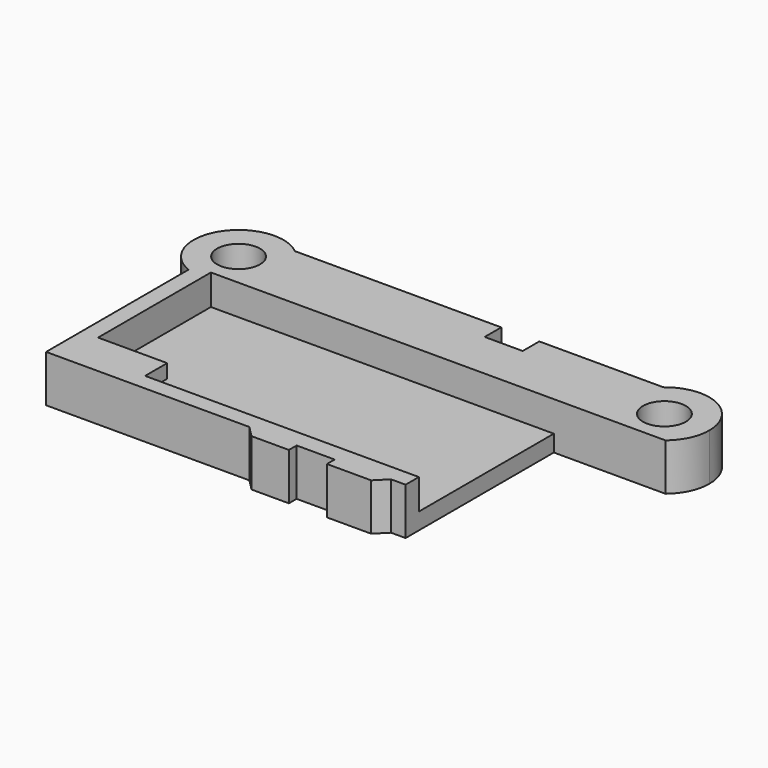
from build123d import *

# Parameters (mm, degrees)
F0_W        = 21.3
F0_H        = 2.5
F0_R        = 1.55
F1_DEPTH    = 3.4
F0_W_2      = 1.2
F0_H_2      = 1.2
F0_W_3      = 3.5
F2_DEPTH    = 3.4
F0_H_3      = 12.2
F3_DEPTH    = 1.2
F4_W        = 5
F4_H        = 1
F5_DEPTH    = 2
F6_T4_DEPTH = 3.4
F6_T9_DEPTH = 3.4


# Not quite as in the source:
# - a fillet or chamfer that OpenCascade refuses, or shapes differently, is made with other operations: its cross-section is extruded or revolved along the edge and cut away or added
# - a feature names something its author has since deleted; it is built from what else it names


with BuildPart() as f1:
    # F0 (on Top) → F1 (new body)
    with BuildSketch(Plane.XY):
        with BuildLine():
            ThreePointArc((-16.4319353276, -0.9810708435), (-15.752751994, 1.4598801321), (-13.6819353276, 0))
            ThreePointArc((-13.6819353276, 0), (-14.1359198167, -1.0960155108), (-15.2319353276, -1.55))
            Line((-15.2319353276, -1.55), (-15.2319353276, -2.5))
            Line((-15.2319353276, -2.5), (-13.1552793618, -2.5))
            ThreePointArc((-13.1552793618, -2.5), (-12.2898585195, -1.3808273084), (-11.9819353276, 0))
            ThreePointArc((-11.9819353276, 0), (-12.2898585195, 1.3808273084), (-13.1552793618, 2.5))
            ThreePointArc((-13.1552793618, 2.5), (-18.0266966766, 1.6588577401), (-16.4319353276, -3.0203476621))
            Line((-16.4319353276, -3.0203476621), (-16.4319353276, -2.5))
            Line((-16.4319353276, -2.5), (-16.4319353276, -0.9810708435))
        make_face()
        with BuildLine():
            ThreePointArc((-15.2319353276, -1.55), (-15.8959534721, -1.4005641377), (-16.4319353276, -0.9810708435))
            Line((-16.4319353276, -0.9810708435), (-16.4319353276, -2.5))
            Line((-16.4319353276, -2.5), (-15.2319353276, -2.5))
            Line((-15.2319353276, -2.5), (-15.2319353276, -1.55))
        make_face()
        with BuildLine():
            ThreePointArc((-11.9819353276, 0), (-12.2898585195, -1.3808273084), (-13.1552793618, -2.5))
            Line((-13.1552793618, -2.5), (-11.7319353276, -2.5))
            Line((-11.7319353276, -2.5), (-11.7319353276, 0))
            Line((-11.7319353276, 0), (-11.9819353276, 0))
        make_face()
        with BuildLine():
            Line((1.7680646724, 2.5), (-13.1552793618, 2.5))
            ThreePointArc((-13.1552793618, 2.5), (-12.2898585195, 1.3808273084), (-11.9819353276, 0))
            Line((-11.9819353276, 0), (-11.7319353276, 0))
            Line((-11.7319353276, 0), (9.5680646724, 0))
            Line((9.5680646724, 0), (9.5680646724, -2.5))
            Line((9.5680646724, -2.5), (13.4914087067, -2.5))
            ThreePointArc((13.4914087067, -2.5), (12.3180646724, 0), (13.4914087067, 2.5))
            Line((13.4914087067, 2.5), (4.5180646724, 2.5))
            Line((4.5180646724, 2.5), (4.5180646724, 1))
            Line((4.5180646724, 1), (1.7680646724, 1))
            Line((1.7680646724, 1), (1.7680646724, 2.5))
        make_face()
        with Locations((-1.0819353276, -1.25)):
            Rectangle(F0_W, F0_H)
        with BuildLine():
            ThreePointArc((13.4914087067, 2.5), (12.3180646724, 0), (13.4914087067, -2.5))
            Line((13.4914087067, -2.5), (17.6447206382, -2.5))
            ThreePointArc((17.6447206382, -2.5), (18.5101414805, -1.3808273084), (18.8180646724, 0))
            ThreePointArc((18.8180646724, 0), (16.9488919809, 2.942076808), (13.4914087067, 2.5))
        make_face()
        with Locations((15.5680646724, 0)):
            Circle(F0_R, mode=Mode.SUBTRACT)
    extrude(amount=F1_DEPTH)

    # F0 (on Top) → F2 (join)
    with BuildSketch(Plane.XY):
        with BuildLine():
            ThreePointArc((-15.2319353276, -3.25), (-15.8428240646, -3.1920706369), (-16.4319353276, -3.0203476621))
            Line((-16.4319353276, -3.0203476621), (-16.4319353276, -14.7))
            Line((-16.4319353276, -14.7), (-15.2319353276, -14.7))
            Line((-15.2319353276, -14.7), (-15.2319353276, -3.25))
        make_face()
        with BuildLine():
            Line((-15.2319353276, -2.5), (-16.4319353276, -2.5))
            Line((-16.4319353276, -2.5), (-16.4319353276, -3.0203476621))
            ThreePointArc((-16.4319353276, -3.0203476621), (-15.8428240646, -3.1920706369), (-15.2319353276, -3.25))
            Line((-15.2319353276, -3.25), (-15.2319353276, -2.5))
        make_face()
        with Locations((-15.8319353276, -15.3)):
            Rectangle(F0_W_2, F0_H_2)
        with Locations((-13.4819353276, -15.3)):
            Rectangle(F0_W_3, F0_H_2)
        Polygon((9.5680646724, -14.7), (-11.7319353276, -14.7), (-11.7319353276, -15.9), (-0.2319353276, -15.9), (7.0180646724, -15.9), (9.5680646724, -15.9), align=None)
        Polygon((7.0180646724, -15.9), (-0.2319353276, -15.9), (-0.2319353276, -16.7), (1.7680646724, -16.7), (1.7680646724, -16), (4.5180646724, -16), (4.5180646724, -16.7), (7.0180646724, -16.7), align=None)
    extrude(amount=F2_DEPTH)

    # F0 (on Top) → F3 (join)
    with BuildSketch(Plane.XY):
        with BuildLine():
            ThreePointArc((-13.1552793618, -2.5), (-14.1279652193, -3.0567548152), (-15.2319353276, -3.25))
            Line((-15.2319353276, -3.25), (-15.2319353276, -14.7))
            Line((-15.2319353276, -14.7), (-11.7319353276, -14.7))
            Line((-11.7319353276, -14.7), (-11.7319353276, -2.5))
            Line((-11.7319353276, -2.5), (-13.1552793618, -2.5))
        make_face()
        with BuildLine():
            Line((-13.1552793618, -2.5), (-15.2319353276, -2.5))
            Line((-15.2319353276, -2.5), (-15.2319353276, -3.25))
            ThreePointArc((-15.2319353276, -3.25), (-14.1279652193, -3.0567548152), (-13.1552793618, -2.5))
        make_face()
        with Locations((-1.0819353276, -8.6)):
            Rectangle(F0_W, F0_H_3)
    extrude(amount=F3_DEPTH)

    # F4 (on face) → F5 (join)
    with BuildSketch(Plane(origin=(0, -14.7, 0), x_dir=(-1, 0, 0), z_dir=(0, 1, 0))):
        with Locations((12.7319353276, 2.9)):
            Rectangle(F4_W, F4_H)
    extrude(amount=F5_DEPTH)

    # F6: chamfer of 1.5 on 2 edges, made by hand


with BuildPart() as f6_tool2:
    # F6_s3 → F6_t4 (new body)
    with BuildSketch(Plane.XY):
        Polygon((-1.7319353276, -15.9), (-0.2319353276, -17.4), (-0.2319353276, -15.9), align=None)
    extrude(amount=F6_T4_DEPTH)

    split(bisect_by=Plane.XZ.offset(16.7), keep=Keep.BOTTOM)


with BuildPart() as f1_1:
    add(f1.part)

    # F6_t1: union F6_tool2
    add(f6_tool2.part)


with BuildPart() as f6_tool7:
    # F6_s8 → F6_t9 (new body)
    with BuildSketch(Plane.XY):
        Polygon((7.0180646724, -17.4), (8.5180646724, -15.9), (7.0180646724, -15.9), align=None)
    extrude(amount=F6_T9_DEPTH)

    split(bisect_by=Plane.XZ.offset(16.7), keep=Keep.BOTTOM)


with BuildPart() as f1_2:
    add(f1_1.part)

    # F6_t6: union F6_tool7
    add(f6_tool7.part)


solid = f1_2.part
